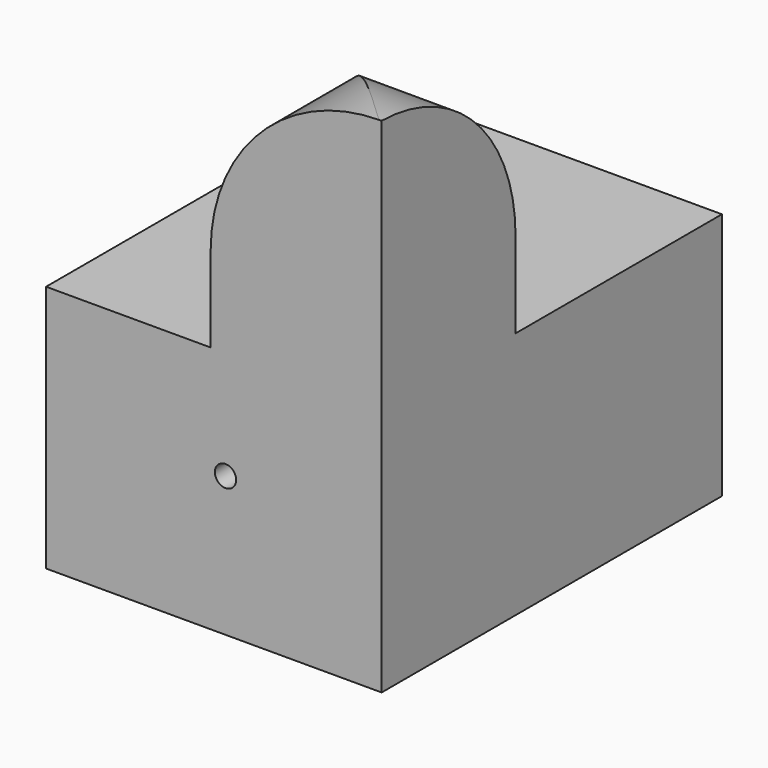
from build123d import *

# Parameters (mm, degrees)
F0_W        = 100.18889606
F0_H        = 74.0776211023
F1_DEPTH    = 127
F2_W        = 51.0549172759
F2_H        = 49.9856282473
F3_DEPTH    = 76.2
F4_T1_DEPTH = 305.0222773169
F4_T3_DEPTH = 303.9856282473
F6_D        = 6.35


# Not quite as in the source:
# - a fillet or chamfer that OpenCascade refuses, or shapes differently, is made with other operations: its cross-section is extruded or revolved along the edge and cut away or added


with BuildPart() as f1:
    # F0 (on Front) → F1 (new body)
    with BuildSketch(Plane.XZ):
        with Locations((50.09444803, 37.0388105512)):
            Rectangle(F0_W, F0_H)
    extrude(amount=F1_DEPTH)

    # F2 (on face) → F3 (join)
    with BuildSketch(Plane.XY.offset(74.0776211023)):
        with Locations((74.661437422, -102.0071858764)):
            Rectangle(F2_W, F2_H)
    extrude(amount=F3_DEPTH)

    # F4: fillet of radius 50.8 on 2 edges, made by hand

    # F4_s2 → F4_t1 (cut)
    with BuildSketch(Plane.YZ.offset(-77.8497012364)):
        with BuildLine():
            ThreePointArc((-77.0143717527, 99.4841490941), (-91.6065681392, 135.1160864184), (-127, 150.2776211023))
            Line((-127, 150.2776211023), (-77.0143717527, 150.2776211023))
            Line((-77.0143717527, 150.2776211023), (-77.0143717527, 99.4841490941))
        make_face()
    extrude(amount=F4_T1_DEPTH, mode=Mode.SUBTRACT)

    # F4_s4 → F4_t3 (cut)
    with BuildSketch(Plane.XZ.offset(-49.9856282473)):
        with BuildLine():
            ThreePointArc((49.1339787841, 99.4776211023), (64.0129542998, 135.3986455866), (99.9339787841, 150.2776211023))
            Line((99.9339787841, 150.2776211023), (49.1339787841, 150.2776211023))
            Line((49.1339787841, 150.2776211023), (49.1339787841, 99.4776211023))
        make_face()
    extrude(amount=F4_T3_DEPTH, mode=Mode.SUBTRACT)

    # F6 (through all)
    with Locations(Plane(origin=(0, 0, 0), x_dir=(-1, 0, 0), z_dir=(0, 1, 0))):
        with Locations((-53.5700023174, 41.735380888)):
            Hole(F6_D / 2)


solid = f1.part
